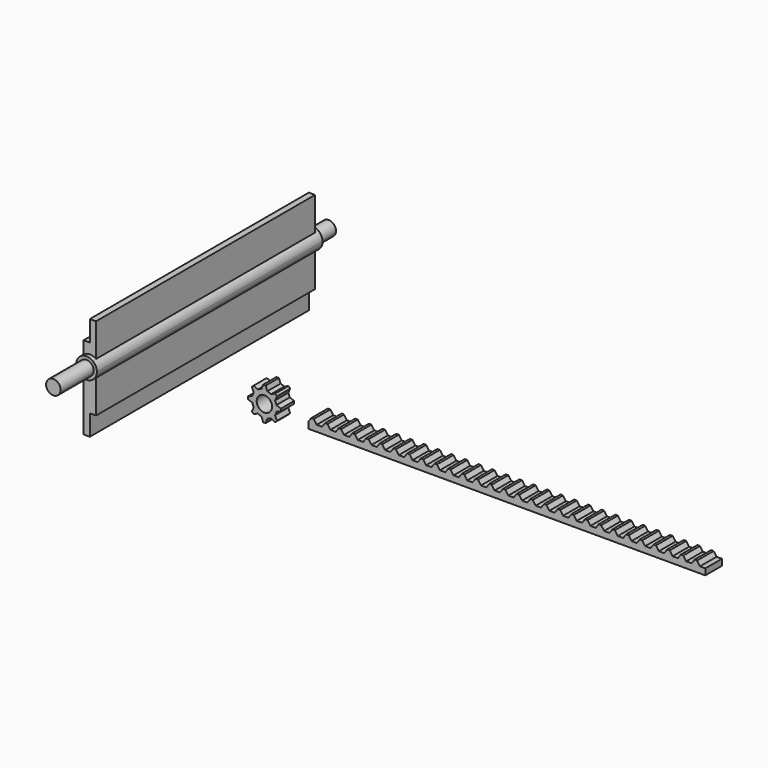
from build123d import *

# Parameters (mm, degrees)
F1_DEPTH      = 33
F2_DEPTH      = 34
F2_DEPTH_BACK = 34
F3_R          = 1.75
F4_DEPTH      = 10
F5_R          = 1.75
F6_DEPTH      = 5
F7_R          = 0.65
F8_DEPTH      = 2
F7_R_2        = 1.85
F9_DEPTH      = 2
F10_DEPTH     = 2.5


with BuildPart() as f1:
    # F0 (on Front) → F1 (new body, symmetric)
    with BuildSketch(Plane.XZ):
        with BuildLine():
            Line((0, 20), (0, 17))
            ThreePointArc((0, 17), (1.5, 17.5), (3, 17))
            Line((3, 17), (3, 25))
            Line((3, 25), (1.5, 25))
            Line((1.5, 25), (1.5, 20))
            Line((1.5, 20), (0, 20))
        make_face()
        with BuildLine():
            Line((0, 13), (0, 0))
            Line((0, 0), (1.5, 0))
            Line((1.5, 0), (1.5, 5))
            Line((1.5, 5), (3, 5))
            Line((3, 5), (3, 13))
            ThreePointArc((3, 13), (1.5, 12.5), (0, 13))
        make_face()
        with BuildLine():
            Line((0, 17), (0, 13))
            ThreePointArc((0, 13), (1.5, 12.5), (3, 13))
            Line((3, 13), (3, 17))
            ThreePointArc((3, 17), (1.5, 17.5), (0, 17))
        make_face()
    extrude(amount=F1_DEPTH, both=True)

    # F0 (on Front) → F2 (join, two sides)
    with BuildSketch(Plane.XZ) as f2_sk:
        with BuildLine():
            Line((0, 17), (0, 13))
            ThreePointArc((0, 13), (1.5, 12.5), (3, 13))
            Line((3, 13), (3, 17))
            ThreePointArc((3, 17), (1.5, 17.5), (0, 17))
        make_face()
        with BuildLine():
            ThreePointArc((0, 17), (-1, 15), (0, 13))
            Line((0, 13), (0, 17))
        make_face()
        with BuildLine():
            Line((3, 17), (3, 13))
            ThreePointArc((3, 13), (3.736068, 13.881966), (4, 15))
            ThreePointArc((4, 15), (3.736068, 16.118034), (3, 17))
        make_face()
    extrude(amount=F2_DEPTH)
    extrude(f2_sk.sketch, amount=-F2_DEPTH_BACK)

    # F3 (on face) → F4 (join)
    with BuildSketch(Plane.XZ.offset(34)):
        with Locations((1.5, 15)):
            Circle(F3_R)
    extrude(amount=F4_DEPTH)

    # F5 (on face) → F6 (join)
    with BuildSketch(Plane(origin=(0, 34, 0), x_dir=(-1, 0, 0), z_dir=(0, 1, 0))):
        with Locations((-1.5, 15)):
            Circle(F5_R)
    extrude(amount=F6_DEPTH)

    # F3 (on face) → F10 (join, symmetric)
    with BuildSketch(Plane.XZ.offset(34)):
        with Locations((1.5, 15)):
            Circle(F3_R)
    extrude(amount=F10_DEPTH, both=True)


with BuildPart() as f8:
    # F7 (on Front) → F8 (new body, symmetric)
    with BuildSketch(Plane.XZ):
        with BuildLine():
            Line((-21.8015, 2.608329), (-21.326647, 1.56779))
            ThreePointArc((-21.326647, 1.56779), (-21.540545, 1.14805), (-21.686097, 0.7))
            Line((-21.686097, 0.7), (-22.757641, 0.3))
            Line((-22.757641, 0.3), (-22.757641, -0.3))
            Line((-22.757641, -0.3), (-21.686097, -0.7))
            ThreePointArc((-21.686097, -0.7), (-21.540545, -1.14805), (-21.326647, -1.56779))
            Line((-21.326647, -1.56779), (-21.8015, -2.608329))
            Line((-21.8015, -2.608329), (-21.377236, -3.032593))
            Line((-21.377236, -3.032593), (-20.336697, -2.55774))
            ThreePointArc((-20.336697, -2.55774), (-19.916957, -2.771639), (-19.468907, -2.91719))
            Line((-19.468907, -2.91719), (-19.068907, -3.988734))
            Line((-19.068907, -3.988734), (-18.468907, -3.988734))
            Line((-18.468907, -3.988734), (-18.068907, -2.91719))
            ThreePointArc((-18.068907, -2.91719), (-17.620856, -2.771639), (-17.201116, -2.55774))
            Line((-17.201116, -2.55774), (-16.160578, -3.032593))
            Line((-16.160578, -3.032593), (-15.736314, -2.608329))
            Line((-15.736314, -2.608329), (-16.211167, -1.56779))
            ThreePointArc((-16.211167, -1.56779), (-15.997268, -1.14805), (-15.851716, -0.7))
            Line((-15.851716, -0.7), (-14.780173, -0.3))
            Line((-14.780173, -0.3), (-14.780173, 0.3))
            Line((-14.780173, 0.3), (-15.851716, 0.7))
            ThreePointArc((-15.851716, 0.7), (-15.997268, 1.14805), (-16.211167, 1.56779))
            Line((-16.211167, 1.56779), (-15.736314, 2.608329))
            Line((-15.736314, 2.608329), (-16.160578, 3.032593))
            Line((-16.160578, 3.032593), (-17.201116, 2.55774))
            ThreePointArc((-17.201116, 2.55774), (-17.620856, 2.771639), (-18.068907, 2.91719))
            Line((-18.068907, 2.91719), (-18.468907, 3.988734))
            Line((-18.468907, 3.988734), (-19.068907, 3.988734))
            Line((-19.068907, 3.988734), (-19.468907, 2.91719))
            ThreePointArc((-19.468907, 2.91719), (-19.916957, 2.771639), (-20.336697, 2.55774))
            Line((-20.336697, 2.55774), (-21.377236, 3.032593))
            Line((-21.377236, 3.032593), (-21.8015, 2.608329))
        make_face()
        with Locations((-18.768907, 0)):
            Circle(F7_R, mode=Mode.SUBTRACT)
    extrude(amount=F8_DEPTH, both=True)


with BuildPart() as f9:
    # F7 (on Front) → F9 (new body, symmetric)
    with BuildSketch(Plane.XZ):
        with BuildLine():
            Line((15.748801, 2.608329), (16.223654, 1.56779))
            ThreePointArc((16.223654, 1.56779), (16.009755, 1.14805), (15.864203, 0.7))
            Line((15.864203, 0.7), (14.79266, 0.3))
            Line((14.79266, 0.3), (14.79266, -0.3))
            Line((14.79266, -0.3), (15.864203, -0.7))
            ThreePointArc((15.864203, -0.7), (16.009755, -1.14805), (16.223654, -1.56779))
            Line((16.223654, -1.56779), (15.748801, -2.608329))
            Line((15.748801, -2.608329), (16.173065, -3.032593))
            Line((16.173065, -3.032593), (17.213603, -2.55774))
            ThreePointArc((17.213603, -2.55774), (17.633343, -2.771639), (18.081394, -2.91719))
            Line((18.081394, -2.91719), (18.481394, -3.988734))
            Line((18.481394, -3.988734), (19.081394, -3.988734))
            Line((19.081394, -3.988734), (19.481394, -2.91719))
            ThreePointArc((19.481394, -2.91719), (19.929444, -2.771639), (20.349184, -2.55774))
            Line((20.349184, -2.55774), (21.389723, -3.032593))
            Line((21.389723, -3.032593), (21.813987, -2.608329))
            Line((21.813987, -2.608329), (21.339134, -1.56779))
            ThreePointArc((21.339134, -1.56779), (21.553032, -1.14805), (21.698584, -0.7))
            Line((21.698584, -0.7), (22.770128, -0.3))
            Line((22.770128, -0.3), (22.770128, 0.3))
            Line((22.770128, 0.3), (21.698584, 0.7))
            ThreePointArc((21.698584, 0.7), (21.553032, 1.14805), (21.339134, 1.56779))
            Line((21.339134, 1.56779), (21.813987, 2.608329))
            Line((21.813987, 2.608329), (21.389723, 3.032593))
            Line((21.389723, 3.032593), (20.349184, 2.55774))
            ThreePointArc((20.349184, 2.55774), (19.929444, 2.771639), (19.481394, 2.91719))
            Line((19.481394, 2.91719), (19.081394, 3.988734))
            Line((19.081394, 3.988734), (18.481394, 3.988734))
            Line((18.481394, 3.988734), (18.081394, 2.91719))
            ThreePointArc((18.081394, 2.91719), (17.633343, 2.771639), (17.213603, 2.55774))
            Line((17.213603, 2.55774), (16.173065, 3.032593))
            Line((16.173065, 3.032593), (15.748801, 2.608329))
        make_face()
        with Locations((18.781394, 0)):
            Circle(F7_R_2, mode=Mode.SUBTRACT)
    extrude(amount=F9_DEPTH, both=True)


with BuildPart() as f10:
    # F7 (on Front) → F10, piece 2 (new body, symmetric)
    with BuildSketch(Plane.XZ):
        Polygon((33.080411, 0), (31.780411, 0), (31.080411, 1), (30.480411, 1), (29.780411, 0), (29.780411, -1.5), (125.480411, -1.5), (125.480411, 0), (124.180411, 0), (123.480411, 1), (122.880411, 1), (122.180411, 0), (120.880411, 0), (120.180411, 1), (119.580411, 1), (118.880411, 0), (117.580411, 0), (116.880411, 1), (116.280411, 1), (115.580411, 0), (114.280411, 0), (113.580411, 1), (112.980411, 1), (112.280411, 0), (110.980411, 0), (110.280411, 1), (109.680411, 1), (108.980411, 0), (107.680411, 0), (106.980411, 1), (106.380411, 1), (105.680411, 0), (104.380411, 0), (103.680411, 1), (103.080411, 1), (102.380411, 0), (101.080411, 0), (100.380411, 1), (99.780411, 1), (99.080411, 0), (97.780411, 0), (97.080411, 1), (96.480411, 1), (95.780411, 0), (94.480411, 0), (93.780411, 1), (93.180411, 1), (92.480411, 0), (91.180411, 0), (90.480411, 1), (89.880411, 1), (89.180411, 0), (87.880411, 0), (87.180411, 1), (86.580411, 1), (85.880411, 0), (84.580411, 0), (83.880411, 1), (83.280411, 1), (82.580411, 0), (81.280411, 0), (80.580411, 1), (79.980411, 1), (79.280411, 0), (77.980411, 0), (77.280411, 1), (76.680411, 1), (75.980411, 0), (74.680411, 0), (73.980411, 1), (73.380411, 1), (72.680411, 0), (71.380411, 0), (70.680411, 1), (70.080411, 1), (69.380411, 0), (68.080411, 0), (67.380411, 1), (66.780411, 1), (66.080411, 0), (64.780411, 0), (64.080411, 1), (63.480411, 1), (62.780411, 0), (61.480411, 0), (60.780411, 1), (60.180411, 1), (59.480411, 0), (58.180411, 0), (57.480411, 1), (56.880411, 1), (56.180411, 0), (54.880411, 0), (54.180411, 1), (53.580411, 1), (52.880411, 0), (51.580411, 0), (50.880411, 1), (50.280411, 1), (49.580411, 0), (48.280411, 0), (47.580411, 1), (46.980411, 1), (46.280411, 0), (44.980411, 0), (44.280411, 1), (43.680411, 1), (42.980411, 0), (41.680411, 0), (40.980411, 1), (40.380411, 1), (39.680411, 0), (38.380411, 0), (37.680411, 1), (37.080411, 1), (36.380411, 0), (35.080411, 0), (34.380411, 1), (33.780411, 1), align=None)
    extrude(amount=F10_DEPTH, both=True)


solid = Compound([f1.part, f8.part, f9.part, f10.part])
